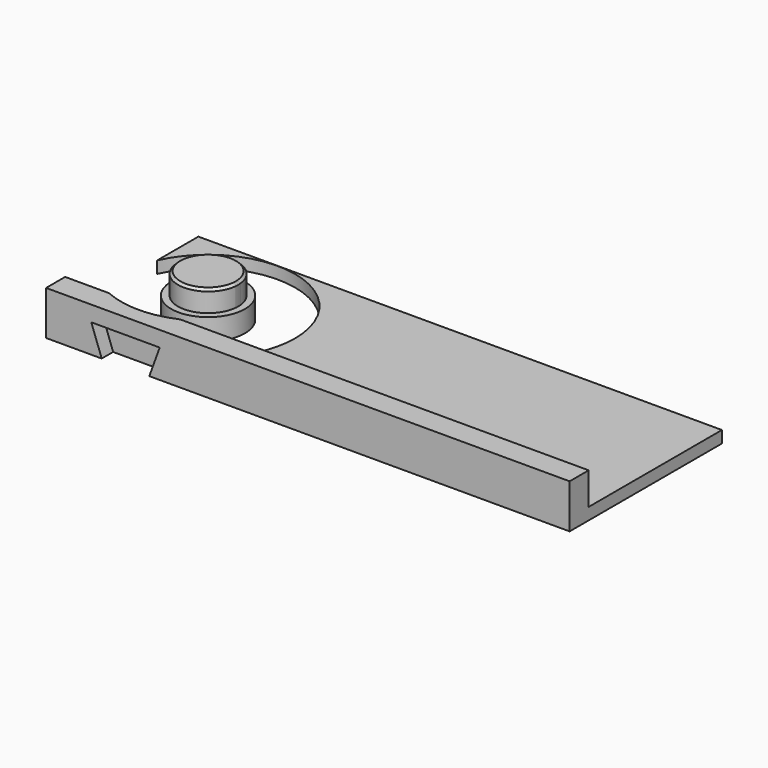
from build123d import *

# Parameters (mm, degrees)
F1_DEPTH = 2.5
F0_R     = 7.75
F2_DEPTH = 4.5
F3_DEPTH = 9
F4_DEPTH = 9.27
F5_SIZE  = 0.5
F8_W     = 10
F8_H     = 6
F9_DEPTH = 3


# Not quite as in the source:
# - a feature of the source that left no trace in its solid (it failed there, or was rolled back) is left out


with BuildPart() as f1:
    # F0 (on Top) → F1 (new body)
    with BuildSketch(Plane.XY):
        with BuildLine():
            Line((55, 18.3124991804), (-55, 18.3124991804))
            Line((-55, 18.3124991804), (-55, 7.4806416837))
            ThreePointArc((-55, 7.4806416837), (-34.4875817002, 17.8830270438), (-20.025, 0))
            ThreePointArc((-20.025, 0), (-22.9626646419, -9.9405840236), (-30.8318583163, -16.6875))
            Line((-30.8318583163, -16.6875), (55, -16.6875))
            Line((55, -16.6875), (55, 18.3124991804))
        make_face()
    extrude(amount=F1_DEPTH)

    # F0 (on Top) → F4 (join)
    with BuildSketch(Plane.XY):
        with BuildLine():
            Line((55, -21.6875008196), (55, -16.6875))
            Line((55, -16.6875), (-30.8318583163, -16.6875))
            ThreePointArc((-30.8318583163, -16.6875), (-38.3125, -18.2875), (-45.7931416837, -16.6875))
            Line((-45.7931416837, -16.6875), (-55, -16.6875))
            Line((-55, -16.6875), (-55, -21.6875008196))
            Line((-55, -21.6875008196), (55, -21.6875008196))
        make_face()
    extrude(amount=F4_DEPTH)

    # F8 (on face) → F9 (cut)
    with BuildSketch(Plane.XZ.offset(21.6875008196)):
        Polygon((-33.3125, 6), (-33.3125, 0), (-31.1286785944, 6), align=None)
        with Locations((-38.3125, 3)):
            Rectangle(F8_W, F8_H)
        Polygon((-45.4963214056, 6), (-43.3125, 0), (-43.3125, 6), align=None)
    extrude(amount=-F9_DEPTH, mode=Mode.SUBTRACT)


with BuildPart() as f2:
    # F0 (on Top) → F2 (new body)
    with BuildSketch(Plane.XY):
        with Locations((-38.3125, 0)):
            Circle(F0_R)
        with BuildLine():
            ThreePointArc((-32.0072938178, 0.5), (-31.9924503917, 0.2501958209), (-31.9875, 0))
            ThreePointArc((-31.9875, 0), (-31.9924503917, -0.2501958209), (-32.0072938178, -0.5))
            ThreePointArc((-32.0072938178, -0.5), (-44.6375, 0), (-32.0072938178, 0.5))
        make_face(mode=Mode.SUBTRACT)
    extrude(amount=F2_DEPTH)


with BuildPart() as f3:
    # F0 (on Top) → F3 (new body)
    with BuildSketch(Plane.XY):
        with BuildLine():
            Line((-32.4964055004, 0.3219779063), (-32.0072938178, 0.5))
            ThreePointArc((-32.0072938178, 0.5), (-44.6375, 0), (-32.0072938178, -0.5))
            Line((-32.0072938178, -0.5), (-32.4964055004, -0.3219779063))
            ThreePointArc((-32.4964055004, -0.3219779063), (-44.1375, 0), (-32.4964055004, 0.3219779063))
        make_face()
        with BuildLine():
            ThreePointArc((-32.0072938178, -0.5), (-31.9924503917, -0.2501958209), (-31.9875, 0))
            ThreePointArc((-31.9875, 0), (-31.9924503917, 0.2501958209), (-32.0072938178, 0.5))
            Line((-32.0072938178, 0.5), (-32.4964055004, 0.3219779063))
            ThreePointArc((-32.4964055004, 0.3219779063), (-32.4897268007, 0.1610505201), (-32.4875, 0))
            ThreePointArc((-32.4875, 0), (-32.4897268007, -0.1610505201), (-32.4964055004, -0.3219779063))
            Line((-32.4964055004, -0.3219779063), (-32.0072938178, -0.5))
        make_face()
        with BuildLine():
            ThreePointArc((-32.4875, 0), (-32.4897268007, 0.1610505201), (-32.4964055004, 0.3219779063))
            ThreePointArc((-32.4964055004, 0.3219779063), (-44.1375, 0), (-32.4964055004, -0.3219779063))
            ThreePointArc((-32.4964055004, -0.3219779063), (-32.4897268007, -0.1610505201), (-32.4875, 0))
        make_face()
    extrude(amount=F3_DEPTH)

    # F5
    f5_edges = [f3.edges().sort_by_distance(p)[0] for p in [
        (-44.617706, 0.5, 9),
    ]]
    chamfer(f5_edges, length=F5_SIZE)


solid = Compound([f1.part, f2.part, f3.part])
